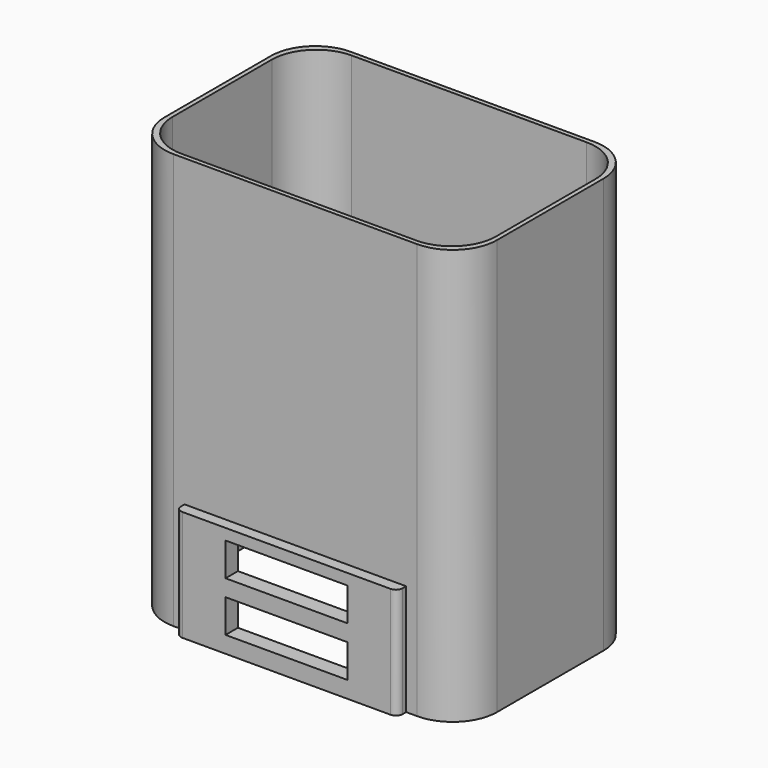
from build123d import *

# Parameters (mm, degrees)
F1_DEPTH    = 20
F0_W        = 58.4
F0_H        = 38.4
F2_DEPTH    = 75
F3_T1_DEPTH = 26
F4_R        = 8
F5_W        = 22
F5_H        = 6
F6_DEPTH    = 3


# Not quite as in the source:
# - a fillet or chamfer that OpenCascade refuses, or shapes differently, is made with other operations: its cross-section is extruded or revolved along the edge and cut away or added


with BuildPart() as f1:
    # F0 (on Top) → F1 (new body)
    with BuildSketch(Plane.XY):
        Polygon((20, -35.6130205363), (20, -33.6130205363), (-20, -33.6130205363), (-20, -35.6130205363), (-10, -35.6130205363), (10, -35.6130205363), align=None)
    extrude(amount=F1_DEPTH)

    # F0 (on Top) → F2 (join)
    with BuildSketch(Plane.XY):
        Polygon((20, -33.6130205363), (30, -33.6130205363), (30, 6.3869794637), (-30, 6.3869794637), (-30, -33.6130205363), (-20, -33.6130205363), align=None)
        with Locations((0, -13.6130205363)):
            Rectangle(F0_W, F0_H, mode=Mode.SUBTRACT)
    extrude(amount=F2_DEPTH)

    # F3: fillet of radius 1.2 on 4 edges, made by hand

    # F3_s2 → F3_t1 (cut)
    with BuildSketch(Plane.XY.offset(-3)):
        with BuildLine():
            ThreePointArc((20, -34.4130205363), (19.6485281374, -35.2615486737), (18.8, -35.6130205363))
            Line((18.8, -35.6130205363), (20, -35.6130205363))
            Line((20, -35.6130205363), (20, -34.4130205363))
        make_face()
        with BuildLine():
            ThreePointArc((-20, -34.4130205363), (-19.6485281374, -35.2615486737), (-18.8, -35.6130205363))
            Line((-18.8, -35.6130205363), (-20, -35.6130205363))
            Line((-20, -35.6130205363), (-20, -34.4130205363))
        make_face()
    extrude(amount=F3_T1_DEPTH, mode=Mode.SUBTRACT)

    # F4
    f4_edges = [f1.edges().sort_by_distance(p)[0] for p in [
        (29.2, 5.586979, 37.5),
        (29.2, -32.813021, 37.5),
        (-29.2, -32.813021, 37.5),
        (-29.2, 5.586979, 37.5),
        (-30, -33.613021, 37.5),
        (-30, 6.386979, 37.5),
        (30, -33.613021, 37.5),
        (30, 6.386979, 37.5),
    ]]
    fillet(f4_edges, radius=F4_R)

    # F5 (on face) → F6 (cut)
    with BuildSketch(Plane.XZ.offset(35.6130205363)):
        with Locations((0, 15)):
            Rectangle(F5_W, F5_H)
        with Locations((0, 6)):
            Rectangle(F5_W, F5_H)
    extrude(amount=-F6_DEPTH, mode=Mode.SUBTRACT)


solid = f1.part
